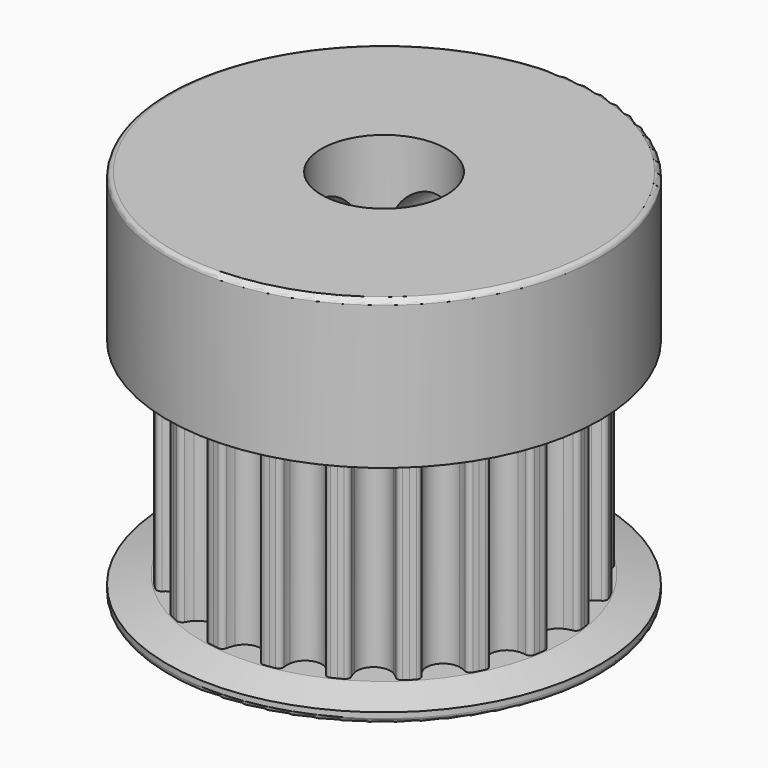
from build123d import *

# Parameters (mm, degrees)
F3_DEPTH    = 5
F4_COUNT    = 20
F5_R        = 11
F6_DEPTH    = 1
F7_R        = 11
F8_DEPTH    = 1
F9_R        = 11
F10_DEPTH   = 7
F11_R       = 3.175
F12_DEPTH   = 19.001
F13_R       = 1.75
F14_DEPTH   = 11.001
F15_R       = 1.75
F16_DEPTH   = 11.0010001
F17_SIZE2   = 0.4689110868
F17_SIZE    = 1.75
F17_2_SIZE2 = 0.4689110868
F17_2_SIZE  = 1.75
F18_R       = 0.25


# Not quite as in the source:
# - a feature names something its author has since deleted; it is built from what else it names


with BuildPart() as f3:
    # F2 (on Top) → F3 (new body, symmetric)
    with BuildSketch(Plane.XY):
        with BuildLine():
            ThreePointArc((0.7733097642, 8.5170606544), (0.459668841, 8.1549092015), (0, 8.0198949053))
            ThreePointArc((0, 8.0198949053), (-0.459668841, 8.1549092015), (-0.7733097642, 8.5170606544))
            ThreePointArc((-0.7733097642, 8.5170606544), (-0.8426497246, 8.6991061844), (-0.8881371246, 8.8885250365))
            ThreePointArc((-0.8881371246, 8.8885250365), (-0.9860029464, 9.0469889833), (-1.1662689318, 9.0938154291))
            ThreePointArc((-1.1662689318, 9.0938154291), (-1.3003949699, 9.0756066024), (-1.4342375717, 9.0554196406))
            Line((-1.4342375717, 9.0554196406), (0, 0))
            Line((0, 0), (1.4342375717, 9.0554196406))
            ThreePointArc((1.4342375717, 9.0554196406), (1.3003949699, 9.0756066024), (1.1662689318, 9.0938154291))
            ThreePointArc((1.1662689318, 9.0938154291), (0.9860029464, 9.0469889833), (0.8881371246, 8.8885250365))
            ThreePointArc((0.8881371246, 8.8885250365), (0.8426497246, 8.6991061844), (0.7733097642, 8.5170606544))
        make_face()
    extrude(amount=F3_DEPTH, both=True)

    # F4: F3 ×20 about axis
    f4_axis = Axis((0, 0, 0), (0, 0, -1))


with BuildPart() as f3_1:
    add(f3.part)
    for i in range(1, F4_COUNT):
        add(f3.part.rotate(f4_axis, i * 360 / F4_COUNT))

    # F5 (on face) → F6 (join)
    with BuildSketch(Plane(origin=(0, 0, -5), x_dir=(1, 0, 0), z_dir=(0, 0, -1))):
        Circle(F5_R)
    extrude(amount=F6_DEPTH)

    # F7 (on face) → F8 (join)
    with BuildSketch(Plane.XY.offset(5)):
        Circle(F7_R)
    extrude(amount=F8_DEPTH)

    # F9 (on face) → F10 (join)
    with BuildSketch(Plane.XY.offset(6)):
        Circle(F9_R)
    extrude(amount=F10_DEPTH)

    # F11 (on face) → F12 (cut, through all)
    with BuildSketch(Plane.XY.offset(13)):
        Circle(F11_R)
    extrude(amount=-F12_DEPTH, mode=Mode.SUBTRACT)

    # F13 (on Front) → F14 (cut, through all)
    with BuildSketch(Plane.XZ):
        with Locations((0, 9)):
            Circle(F13_R)
    extrude(amount=-F14_DEPTH, mode=Mode.SUBTRACT)

    # F15 (on Right) → F16 (cut, through all)
    with BuildSketch(Plane.YZ):
        with Locations((0, 9)):
            Circle(F15_R)
    extrude(amount=-F16_DEPTH, mode=Mode.SUBTRACT)

    # F17
    f17_edges = [f3_1.edges().sort_by_distance(p)[0] for p in [
        (-11, 0, -5),
    ]]
    f17_side = f3_1.faces().sort_by_distance((-10.688873, 0, -5))[0]
    chamfer(f17_edges, length=F17_SIZE, length2=F17_SIZE2, reference=f17_side)

    # F17#2
    f17_2_edges = [f3_1.edges().sort_by_distance(p)[0] for p in [
        (-11, 0, 5),
    ]]
    f17_2_side = f3_1.faces().sort_by_distance((-10.688873, 0, 5))[0]
    chamfer(f17_2_edges, length=F17_2_SIZE, length2=F17_2_SIZE2, reference=f17_2_side)

    # F18
    f18_edges = [f3_1.edges().sort_by_distance(p)[0] for p in [
        (-11, 0, 13),
        (-11, 0, -6),
    ]]
    fillet(f18_edges, radius=F18_R)


solid = f3_1.part
